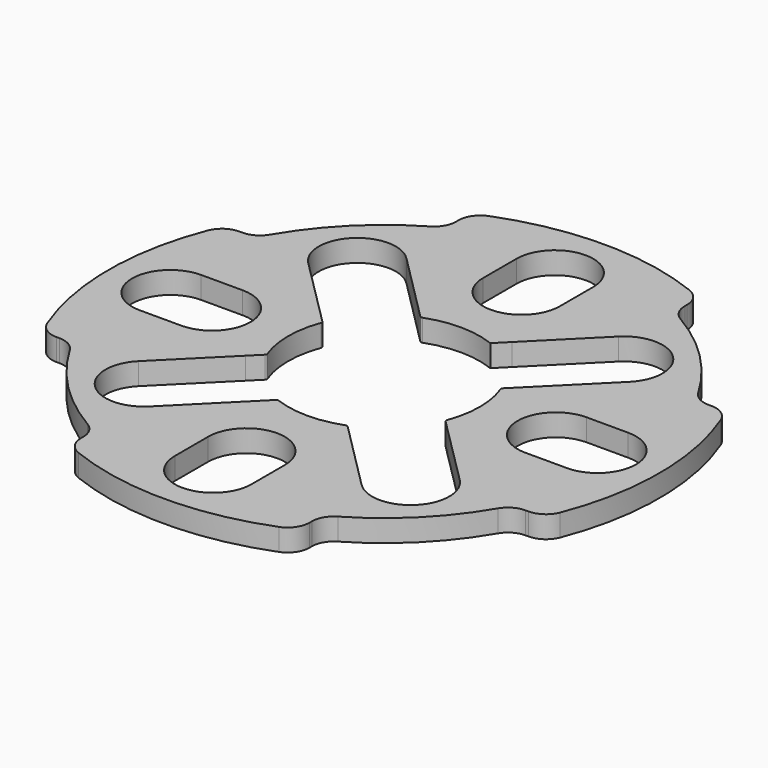
from build123d import *

# Parameters (mm, degrees)
F1_DEPTH = 1


# Not quite as in the source:
# - ends of sketch curves that miss each other by under 0.0002 mm in the source are joined


with BuildPart() as f1:
    # F0 (on Top) → F1 (new body)
    with BuildSketch(Plane.XY):
        with BuildLine():
            ThreePointArc((5.1893277963, 10.709786768), (5.015248305, 11.2735733528), (4.5536171698, 11.6410725739))
            ThreePointArc((4.5536171698, 11.6410725739), (0, 12.5), (-4.5536171698, 11.6410725739))
            ThreePointArc((-4.5536171698, 11.6410725739), (-5.015248305, 11.2735733528), (-5.1893277963, 10.709786768))
            Line((-5.1893277963, 10.709786768), (-5.1893277963, 10.5791593824))
            ThreePointArc((-5.1893277963, 10.5791593824), (-5.3218672589, 10.0816533863), (-5.6843522286, 9.716025745))
            ThreePointArc((-5.6843522286, 9.716025745), (-7.9596801612, 7.9596801612), (-9.716025745, 5.6843522286))
            ThreePointArc((-9.716025745, 5.6843522286), (-10.0816533863, 5.3218672589), (-10.5791593824, 5.1893277963))
            Line((-10.5791593824, 5.1893277963), (-10.709786768, 5.1893277963))
            ThreePointArc((-10.709786768, 5.1893277963), (-11.2735733528, 5.015248305), (-11.6410725739, 4.5536171698))
            ThreePointArc((-11.6410725739, 4.5536171698), (-12.5, 0), (-11.6410725739, -4.5536171698))
            ThreePointArc((-11.6410725739, -4.5536171698), (-11.2735733528, -5.015248305), (-10.709786768, -5.1893277963))
            Line((-10.709786768, -5.1893277963), (-10.5791593824, -5.1893277963))
            ThreePointArc((-10.5791593824, -5.1893277963), (-10.0816533863, -5.3218672589), (-9.716025745, -5.6843522286))
            ThreePointArc((-9.716025745, -5.6843522286), (-7.9596801612, -7.9596801612), (-5.6843522286, -9.716025745))
            ThreePointArc((-5.6843522286, -9.716025745), (-5.3218672589, -10.0816533863), (-5.1893277963, -10.5791593824))
            Line((-5.1893277963, -10.5791593824), (-5.1893277963, -10.709786768))
            ThreePointArc((-5.1893277963, -10.709786768), (-5.015248305, -11.2735733528), (-4.5536171698, -11.6410725739))
            ThreePointArc((-4.5536171698, -11.6410725739), (0, -12.5), (4.5536171698, -11.6410725739))
            ThreePointArc((4.5536171698, -11.6410725739), (5.015248305, -11.2735733528), (5.1893277963, -10.709786768))
            Line((5.1893277963, -10.709786768), (5.1893277963, -10.5791593824))
            ThreePointArc((5.1893277963, -10.5791593824), (5.3218672589, -10.0816533863), (5.6843522286, -9.716025745))
            ThreePointArc((5.6843522286, -9.716025745), (7.9596801612, -7.9596801612), (9.716025745, -5.6843522286))
            ThreePointArc((9.716025745, -5.6843522286), (10.0816533863, -5.3218672589), (10.5791593824, -5.1893277963))
            Line((10.5791593824, -5.1893277963), (10.709786768, -5.1893277963))
            ThreePointArc((10.709786768, -5.1893277963), (11.2735733528, -5.015248305), (11.6410725739, -4.5536171698))
            ThreePointArc((11.6410725739, -4.5536171698), (12.5, 0), (11.6410725739, 4.5536171698))
            ThreePointArc((11.6410725739, 4.5536171698), (11.2735733528, 5.015248305), (10.709786768, 5.1893277963))
            Line((10.709786768, 5.1893277963), (10.5791593824, 5.1893277963))
            ThreePointArc((10.5791593824, 5.1893277963), (10.0816533863, 5.3218672589), (9.716025745, 5.6843522286))
            ThreePointArc((9.716025745, 5.6843522286), (7.9596801612, 7.9596801612), (5.6843522286, 9.716025745))
            ThreePointArc((5.6843522286, 9.716025745), (5.3218672589, 10.0816533863), (5.1893277963, 10.5791593824))
            Line((5.1893277963, 10.5791593824), (5.1893277963, 10.709786768))
        make_face()
        with BuildLine():
            Line((-1.7389636828, -9.696227699), (-1.7389636828, -7.803772301))
            ThreePointArc((-1.7389636828, -7.803772301), (0, -6.0648086182), (1.7389636828, -7.803772301))
            Line((1.7389636828, -7.803772301), (1.7389636828, -9.696227699))
            ThreePointArc((1.7389636828, -9.696227699), (0, -11.4351913818), (-1.7389636828, -9.696227699))
        make_face(mode=Mode.SUBTRACT)
        with BuildLine():
            Line((-4.0980324058, 1.6278386791), (-4.596886989, 2.1259958547))
            Line((-4.596886989, 2.1259958547), (-7.2887076389, 4.8140532918))
            ThreePointArc((-7.2887076389, 4.8140532918), (-7.2895746597, 7.2895734489), (-4.8140532909, 7.2887076381))
            Line((-4.8140532909, 7.2887076381), (-2.1259958547, 4.596886989))
            Line((-2.1259958547, 4.596886989), (-1.6278386791, 4.0980324058))
            ThreePointArc((-1.6278386791, 4.0980324058), (-1.5783462567, 4.0709813489), (-1.5220880269, 4.0750150967))
            ThreePointArc((-1.5220880269, 4.0750150967), (0.0320676528, 4.349881799), (1.5820019575, 4.052131514))
            Line((1.5820019575, 4.052131514), (2.1259958547, 4.596886989))
            Line((2.1259958547, 4.596886989), (4.8140532909, 7.2887076381))
            ThreePointArc((4.8140532909, 7.2887076381), (7.2895746597, 7.2895734489), (7.2887088489, 4.8140520801))
            Line((7.2887088489, 4.8140520801), (4.596886989, 2.1259958547))
            Line((4.596886989, 2.1259958547), (4.0980324058, 1.6278386791))
            ThreePointArc((4.0980324058, 1.6278386791), (4.0709813489, 1.5783462567), (4.0750150967, 1.5220880269))
            ThreePointArc((4.0750150967, 1.5220880269), (4.35, 0), (4.0750150967, -1.5220880269))
            ThreePointArc((4.0750150967, -1.5220880269), (4.0709813489, -1.5783462567), (4.0980324058, -1.6278386791))
            Line((4.0980324058, -1.6278386791), (4.596886989, -2.1259958547))
            Line((4.596886989, -2.1259958547), (7.2887076389, -4.8140532918))
            ThreePointArc((7.2887076389, -4.8140532918), (7.2904398646, -7.2887076385), (4.8157843062, -7.2904386534))
            Line((4.8157843062, -7.2904386534), (4.8140532909, -7.2887076381))
            Line((4.8140532909, -7.2887076381), (2.1259958547, -4.596886989))
            Line((2.1259958547, -4.596886989), (1.6278386791, -4.0980324058))
            ThreePointArc((1.6278386791, -4.0980324058), (1.5783462567, -4.0709813489), (1.5220880269, -4.0750150967))
            ThreePointArc((1.5220880269, -4.0750150967), (0, -4.35), (-1.5220880269, -4.0750150967))
            ThreePointArc((-1.5220880269, -4.0750150967), (-1.5783462567, -4.0709813489), (-1.6278386791, -4.0980324058))
            Line((-1.6278386791, -4.0980324058), (-2.1259958547, -4.596886989))
            Line((-2.1259958547, -4.596886989), (-4.8140532909, -7.2887076381))
            ThreePointArc((-4.8140532909, -7.2887076381), (-7.2895746597, -7.2895734489), (-7.2887088489, -4.8140520801))
            Line((-7.2887088489, -4.8140520801), (-4.596886989, -2.1259958547))
            Line((-4.596886989, -2.1259958547), (-4.0980324058, -1.6278386791))
            ThreePointArc((-4.0980324058, -1.6278386791), (-4.0709813489, -1.5783462567), (-4.0750150967, -1.5220880269))
            ThreePointArc((-4.0750150967, -1.5220880269), (-4.35, 0), (-4.0750150967, 1.5220880269))
            ThreePointArc((-4.0750150967, 1.5220880269), (-4.0709813489, 1.5783462567), (-4.0980324058, 1.6278386791))
        make_face(mode=Mode.SUBTRACT)
        with BuildLine():
            Line((-7.803772301, -1.7389636828), (-9.696227699, -1.7389636828))
            ThreePointArc((-9.696227699, -1.7389636828), (-11.4351913818, 0), (-9.696227699, 1.7389636828))
            Line((-9.696227699, 1.7389636828), (-7.803772301, 1.7389636828))
            ThreePointArc((-7.803772301, 1.7389636828), (-6.0648086182, 0), (-7.803772301, -1.7389636828))
        make_face(mode=Mode.SUBTRACT)
        with BuildLine():
            Line((9.696227699, -1.7389636828), (7.803772301, -1.7389636828))
            ThreePointArc((7.803772301, -1.7389636828), (6.0648086182, 0), (7.803772301, 1.7389636828))
            Line((7.803772301, 1.7389636828), (9.696227699, 1.7389636828))
            ThreePointArc((9.696227699, 1.7389636828), (11.4351913818, 0), (9.696227699, -1.7389636828))
        make_face(mode=Mode.SUBTRACT)
        with BuildLine():
            Line((1.7389636828, 9.696227699), (1.7389636828, 7.803772301))
            ThreePointArc((1.7389636828, 7.803772301), (0, 6.0648086182), (-1.7389636828, 7.803772301))
            Line((-1.7389636828, 7.803772301), (-1.7389636828, 9.696227699))
            ThreePointArc((-1.7389636828, 9.696227699), (0, 11.4351913818), (1.7389636828, 9.696227699))
        make_face(mode=Mode.SUBTRACT)
    extrude(amount=F1_DEPTH)


solid = f1.part
